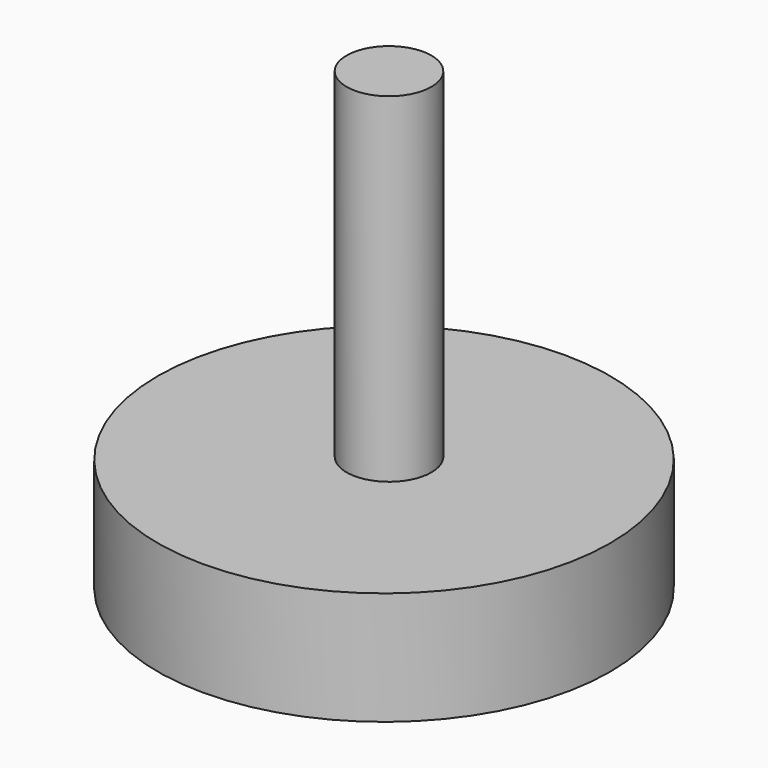
from build123d import *

# Parameters (mm, degrees)
F0_R     = 12.7
F1_DEPTH = 6.35
F2_R     = 2.38125
F3_DEPTH = 25.4


# Not quite as in the source:
# - a length typed as a fraction of an inch, garbled in the dataset ("3 / 203.2 mm" for 3/8 in), is restored


with BuildPart() as f1:
    # F0 (on Top) → F1 (new body)
    with BuildSketch(Plane.XY):
        Circle(F0_R)
    extrude(amount=F1_DEPTH)

    # F2 (on Top) → F3 (join)
    with BuildSketch(Plane.XY):
        with Locations((0, 0.3521142062)):
            Circle(F2_R)
    extrude(amount=F3_DEPTH)


solid = f1.part
